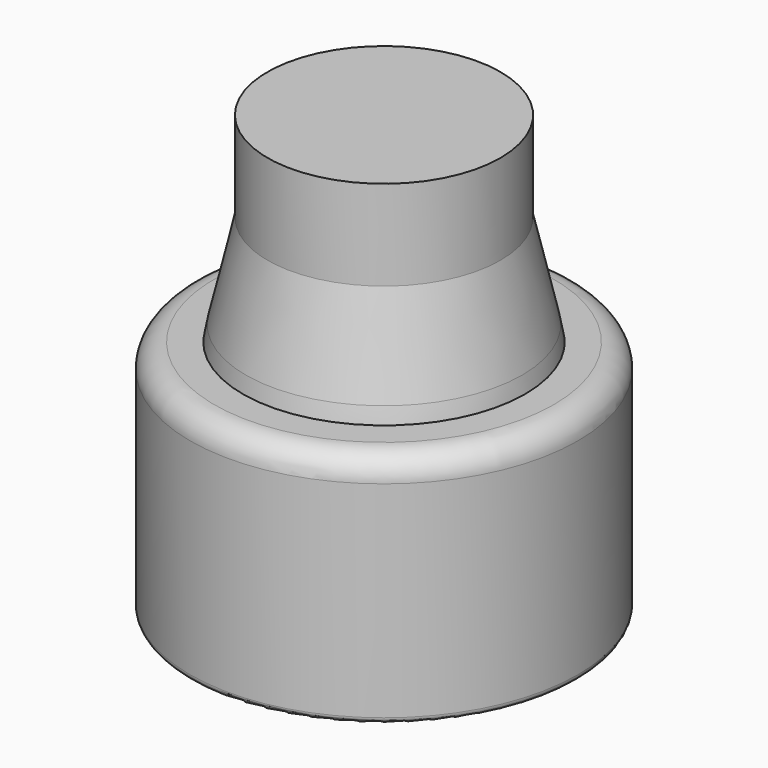
from build123d import *

# Parameters (mm, degrees)
F2_R     = 3.613048962
F3_DEPTH = 7.85
F4_R     = 3.375
F5_DEPTH = 1
F5_TAPER = 70


# Not quite as in the source:
# - an extrude ends at something that could not be found from the text; its depth is read off the source's solid


with BuildPart() as f1:
    # F0 (on Front) → F1 (revolve)
    with BuildSketch(Plane.XZ):
        with BuildLine():
            Line((5.65, 7.85), (3.375, 7.85))
            Line((3.375, 7.85), (3.375, 4.75))
            Line((3.375, 4.75), (1.25, 3.523130678))
            Line((1.25, 3.523130678), (0, 3.523130678))
            Line((0, 3.523130678), (0, 0))
            Line((0, 0), (6.25, 0))
            ThreePointArc((6.25, 0), (6.3914213562, 0.0585786438), (6.45, 0.2))
            Line((6.45, 0.2), (6.45, 7.05))
            ThreePointArc((6.45, 7.05), (6.2156854249, 7.6156854249), (5.65, 7.85))
        make_face()
    revolve(axis=Axis((0, 0, 1.761565339), (0, 0, -1)))

    # F2 (on face) → F3 (join, through all)
    with BuildSketch(Plane.XY.offset(7.85)):
        Circle(F2_R)
        with BuildLine():
            ThreePointArc((-0.6519999327, 2.8747028554), (0, 3.375), (0.6519999327, 2.8747028554))
            Line((0.6519999327, 2.8747028554), (0.6657660801, 2.8233268939))
            ThreePointArc((0.6657660801, 2.8233268939), (1.216024481, 2.1062161843), (2.1121897733, 1.9882337853))
            Line((2.1121897733, 1.9882337853), (2.1635657348, 2.0019999327))
            ThreePointArc((2.1635657348, 2.0019999327), (2.9228357378, 1.6875), (2.8155656675, 0.8727029227))
            Line((2.8155656675, 0.8727029227), (2.7779558534, 0.8350931086))
            ThreePointArc((2.7779558534, 0.8350931086), (2.432048962, 0), (2.7779558534, -0.8350931086))
            Line((2.7779558534, -0.8350931086), (2.8155656675, -0.8727029227))
            ThreePointArc((2.8155656675, -0.8727029227), (2.9228357378, -1.6875), (2.1635657348, -2.0019999327))
            Line((2.1635657348, -2.0019999327), (2.1121897733, -1.9882337853))
            ThreePointArc((2.1121897733, -1.9882337853), (1.216024481, -2.1062161843), (0.6657660801, -2.8233268939))
            Line((0.6657660801, -2.8233268939), (0.6519999327, -2.8747028554))
            ThreePointArc((0.6519999327, -2.8747028554), (0, -3.375), (-0.6519999327, -2.8747028554))
            Line((-0.6519999327, -2.8747028554), (-0.6657660801, -2.8233268939))
            ThreePointArc((-0.6657660801, -2.8233268939), (-1.216024481, -2.1062161843), (-2.1121897733, -1.9882337853))
            Line((-2.1121897733, -1.9882337853), (-2.1635657348, -2.0019999327))
            ThreePointArc((-2.1635657348, -2.0019999327), (-2.9228357378, -1.6875), (-2.8155656675, -0.8727029227))
            Line((-2.8155656675, -0.8727029227), (-2.7779558534, -0.8350931086))
            ThreePointArc((-2.7779558534, -0.8350931086), (-2.432048962, 0), (-2.7779558534, 0.8350931086))
            Line((-2.7779558534, 0.8350931086), (-2.8155656675, 0.8727029227))
            ThreePointArc((-2.8155656675, 0.8727029227), (-2.9228357378, 1.6875), (-2.1635657348, 2.0019999327))
            Line((-2.1635657348, 2.0019999327), (-2.1121897733, 1.9882337853))
            ThreePointArc((-2.1121897733, 1.9882337853), (-1.216024481, 2.1062161843), (-0.6657660801, 2.8233268939))
            Line((-0.6657660801, 2.8233268939), (-0.6519999327, 2.8747028554))
        make_face(mode=Mode.SUBTRACT)
    extrude(amount=-F3_DEPTH)

    # F4 (on face) → F5 (cut)
    with BuildSketch(Plane.XY.offset(7.85)):
        Circle(F4_R)
    extrude(amount=-F5_DEPTH, taper=F5_TAPER, mode=Mode.SUBTRACT)


with BuildPart() as f7:
    # F6 (on Front) → F7 (revolve)
    with BuildSketch(Plane.XZ):
        with BuildLine():
            Line((3.875, 14.5), (0, 14.5))
            Line((0, 14.5), (0, 0))
            Line((0, 0), (3.495, 0))
            Line((3.495, 0), (4.5970197549, 4.7733719814))
            ThreePointArc((4.5970197549, 4.7733719814), (4.8020592366, 6.5729804161), (4.5970197549, 8.3725888509))
            Line((4.5970197549, 8.3725888509), (3.875, 11.5))
            Line((3.875, 11.5), (3.875, 14.5))
        make_face()
    revolve(axis=Axis((0, 0, 7.25), (0, 0, -1)))


with BuildPart() as f9:
    # F8 (on Front) → F9 (revolve)
    with BuildSketch(Plane.XZ):
        with BuildLine():
            Line((0, 7.3151008031), (0, 0))
            Line((0, 0), (5.4641815853, 0))
            ThreePointArc((5.4641815853, 0), (5.8051807653, 0.1343231492), (5.9629636104, 0.4651217631))
            Line((5.9629636104, 0.4651217631), (6.3226162816, 5.6083945828))
            ThreePointArc((6.3226162816, 5.6083945828), (6.3215840066, 6.4599817167), (6.2, 7.3028453127))
            ThreePointArc((6.2, 7.3028453127), (6.0352373223, 7.577508433), (5.7376039765, 7.6958340895))
            Line((5.7376039765, 7.6958340895), (3.75, 7.8))
            Line((3.75, 7.8), (1, 7.3151008031))
            Line((1, 7.3151008031), (0, 7.3151008031))
        make_face()
    revolve(axis=Axis((0, 0, 3.6575504015), (0, 0, 1)))


solid = Compound([f1.part, f7.part, f9.part])
